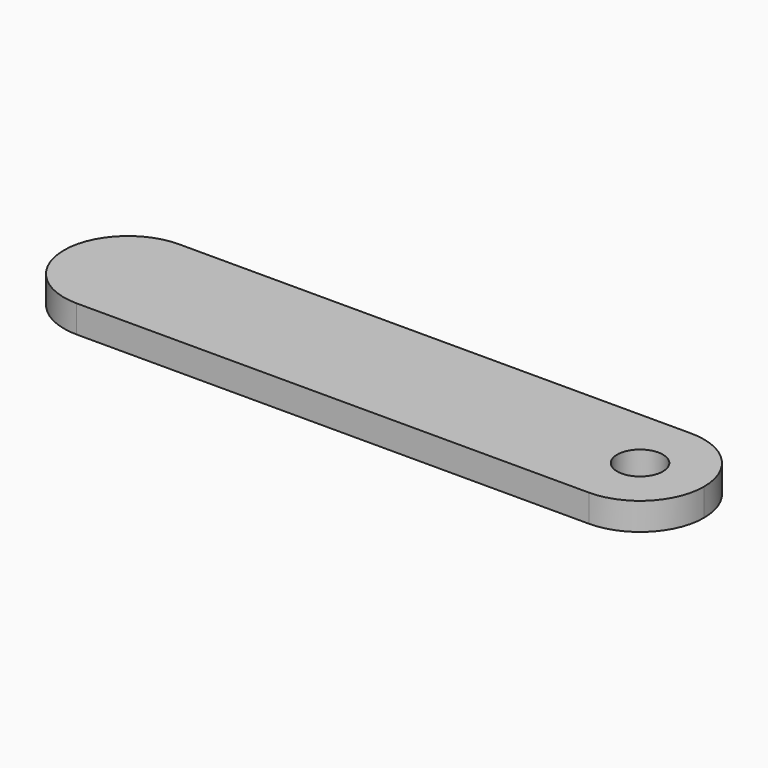
from build123d import *

# Parameters (mm, degrees)
F0_W     = 70
F0_H     = 14
F0_R     = 2.5
F1_DEPTH = 3
F2_R     = 6.99999


# Not quite as in the source:
# - a fillet or chamfer is up to 0.001 mm smaller than in the source, because OpenCascade refuses the exact size


with BuildPart() as f1:
    # F0 (on Top) → F1 (new body)
    with BuildSketch(Plane.XY):
        Rectangle(F0_W, F0_H)
        with Locations((28, 0)):
            Circle(F0_R, mode=Mode.SUBTRACT)
    extrude(amount=F1_DEPTH)

    # F2 (radius 7 in the source; OpenCascade refuses exactly that, so slightly less here)
    f2_edges = [f1.edges().sort_by_distance(p)[0] for p in [
        (35, 7, 1.5),
        (35, -7, 1.5),
        (-35, -7, 1.5),
        (-35, 7, 1.5),
    ]]
    fillet(f2_edges, radius=F2_R)


solid = f1.part
